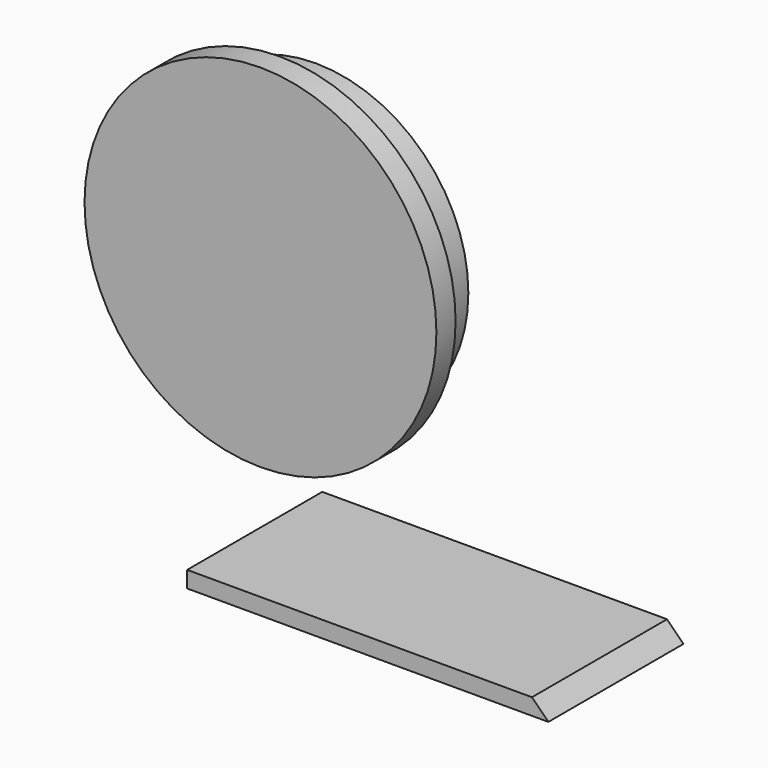
from build123d import *

# Parameters (mm, degrees)
F0_W        = 74.4691416621
F0_H        = 33.9839337394
F1_DEPTH    = 3.302
F2_R        = 35.4048098896
F3_DEPTH    = 4.826
F4_T1_DEPTH = 60.1122328971
F5_R        = 30.7241167349
F6_DEPTH    = 9.144


# Not quite as in the source:
# - a fillet or chamfer that OpenCascade refuses, or shapes differently, is made with other operations: its cross-section is extruded or revolved along the edge and cut away or added


with BuildPart() as f1:
    # F0 (on Top) → F1 (new body)
    with BuildSketch(Plane.XY):
        with Locations((1.2559294701, -1.4781397767)):
            Rectangle(F0_W, F0_H)
    extrude(amount=F1_DEPTH)

    # F4: chamfer of 5.08 on 1 edges, made by hand

    # F4_s2 → F4_t1 (cut)
    with BuildSketch(Plane.XZ.offset(-28.5779766718)):
        Polygon((38.4905003011, -1.778), (33.4105003011, 3.302), (38.4905003011, 3.302), align=None)
    extrude(amount=F4_T1_DEPTH, mode=Mode.SUBTRACT)


with BuildPart() as f3:
    # F2 (on Front) → F3 (new body)
    with BuildSketch(Plane.XZ):
        with Locations((-32.1369804442, 52.6006408036)):
            Circle(F2_R)
    extrude(amount=F3_DEPTH)


with BuildPart() as f6:
    # F5 (on Front) → F6 (new body)
    with BuildSketch(Plane.XZ):
        with Locations((-54.0490671992, 78.4981995821)):
            Circle(F5_R)
    extrude(amount=-F6_DEPTH)


with BuildPart() as f6_1:
    # F7: moved
    add(f6.part.moved(Location((21.844, 0, -26.162))))


solid = Compound([f1.part, f3.part, f6_1.part])
